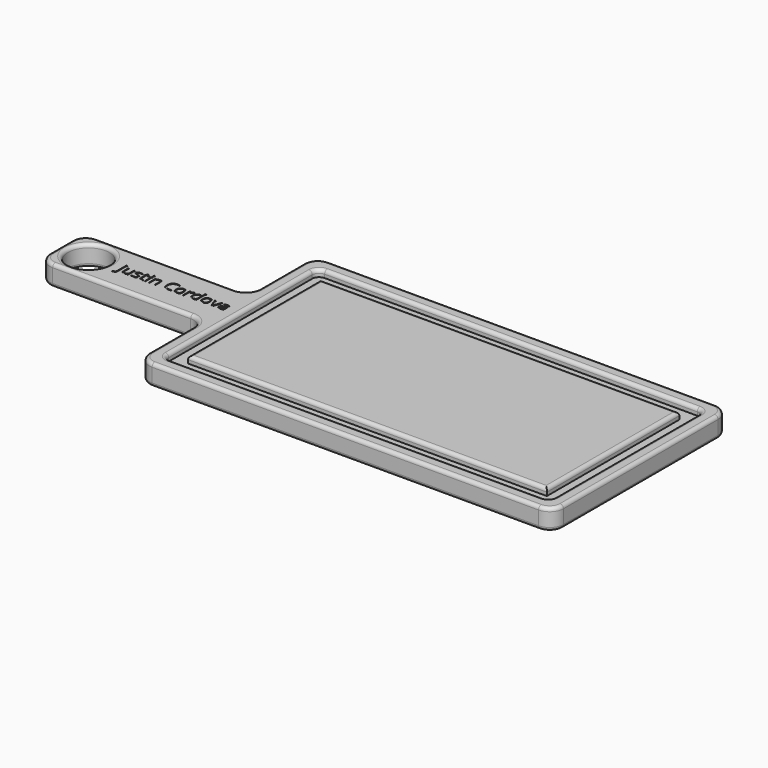
from build123d import *

# Parameters (mm, degrees)
F0_W         = 152.4
F0_H         = 50.8
F1_DEPTH     = 19.05
F2_R         = 19.05
F3_DEPTH     = 25.4
F5_DEPTH     = 6.35
F6_R         = 6.35
F7_R         = 12.7
F8_R         = 3.17499
F9_TEXT_SIZE = 14.9048732407
F10_DEPTH    = 0.508


# Not quite as in the source:
# - a fillet or chamfer is up to 0.001 mm smaller than in the source, because OpenCascade refuses the exact size
# - Text() gives the source's letters only with a copy of the font that has no kerning and outlines rounded to 1/6400 em; it was checked with that copy


with BuildPart() as f1:
    # F0 (on Top) → F1 (new body)
    with BuildSketch(Plane.XY):
        Polygon((0, 76.2), (0, 0), (381, 0), (381, 203.2), (0, 203.2), (0, 127), align=None)
        with Locations((-76.2, 101.6)):
            Rectangle(F0_W, F0_H)
    extrude(amount=F1_DEPTH)

    # F2 (on face) → F3 (cut)
    with BuildSketch(Plane.XY.offset(19.05)):
        with Locations((-127, 101.6)):
            Circle(F2_R)
    extrude(amount=-F3_DEPTH, mode=Mode.SUBTRACT)

    # F4 (on face) → F5 (cut)
    with BuildSketch(Plane.XY.offset(19.05)):
        Polygon((12.6999939203, 76.2), (12.6999939203, 12.6999939203), (368.3000060797, 12.6999939203), (368.3000060797, 190.5000060797), (12.6999939203, 190.5000060797), (12.6999939203, 127), align=None)
        Polygon((25.4000002861, 76.2), (25.4000002861, 127), (25.4000002861, 177.7999997139), (355.5999997139, 177.7999997139), (355.5999997139, 25.4000002861), (25.4000002861, 25.4000002861), align=None, mode=Mode.SUBTRACT)
    extrude(amount=-F5_DEPTH, mode=Mode.SUBTRACT)

    # F6
    f6_edges = [f1.edges().sort_by_distance(p)[0] for p in [
        (368.300006, 12.699994, 15.875),
        (12.699994, 12.699994, 15.875),
        (12.699994, 190.500006, 15.875),
        (368.300006, 190.500006, 15.875),
    ]]
    fillet(f6_edges, radius=F6_R)

    # F7
    f7_edges = [f1.edges().sort_by_distance(p)[0] for p in [
        (0, 0, 9.525),
        (0, 203.2, 9.525),
        (-152.4, 127, 9.525),
        (-152.4, 76.2, 9.525),
        (381, 203.2, 9.525),
        (381, 0, 9.525),
        (0, 76.2, 9.525),
        (0, 127, 9.525),
    ]]
    fillet(f7_edges, radius=F7_R)

    # F8 (radius 3.175 in the source; OpenCascade refuses exactly that, so slightly less here)
    f8_edges = [f1.edges().sort_by_distance(p)[0] for p in [
        (190.5, 177.8, 19.05),
        (355.6, 101.6, 19.05),
        (190.5, 25.4, 19.05),
        (25.4, 101.6, 19.05),
        (0, 38.1, 19.05),
        (-3.719744, 72.480256, 19.05),
        (3.719744, 3.719744, 19.05),
        (-76.2, 76.2, 19.05),
        (190.5, 0, 19.05),
        (-148.680256, 79.919744, 19.05),
        (377.280256, 3.719744, 19.05),
        (-152.4, 101.6, 19.05),
        (381, 101.6, 19.05),
        (-148.680256, 123.280256, 19.05),
        (377.280256, 199.480256, 19.05),
        (-76.2, 127, 19.05),
        (190.5, 203.2, 19.05),
        (-3.719744, 130.719744, 19.05),
        (3.719744, 199.480256, 19.05),
        (0, 165.1, 19.05),
        (190.5, 12.699994, 19.05),
        (14.559866, 14.559866, 19.05),
        (366.440134, 14.559866, 19.05),
        (12.699994, 101.6, 19.05),
        (368.300006, 101.6, 19.05),
        (14.559866, 188.640134, 19.05),
        (366.440134, 188.640134, 19.05),
        (190.5, 190.500006, 19.05),
        (-146.05, 101.6, 19.05),
        (0, 38.1, 0),
        (-3.719744, 72.480256, 0),
        (3.719744, 3.719744, 0),
        (-76.2, 76.2, 0),
        (190.5, 0, 0),
        (-148.680256, 79.919744, 0),
        (377.280256, 3.719744, 0),
        (-152.4, 101.6, 0),
        (381, 101.6, 0),
        (-148.680256, 123.280256, 0),
        (377.280256, 199.480256, 0),
        (-76.2, 127, 0),
        (190.5, 203.2, 0),
        (-3.719744, 130.719744, 0),
        (3.719744, 199.480256, 0),
        (0, 165.1, 0),
        (-146.05, 101.6, 0),
    ]]
    fillet(f8_edges, radius=F8_R)

    # F9 (on face) → F10 (cut)
    with BuildSketch(Plane.XY.offset(19.05)):
        with Locations((-98.1473965449, 96.5930839211)):
            Text('Justin Cordova', F9_TEXT_SIZE, font='Open Sans', text_align=(TextAlign.LEFT, TextAlign.BOTTOM))
    extrude(amount=-F10_DEPTH, mode=Mode.SUBTRACT)


solid = f1.part
